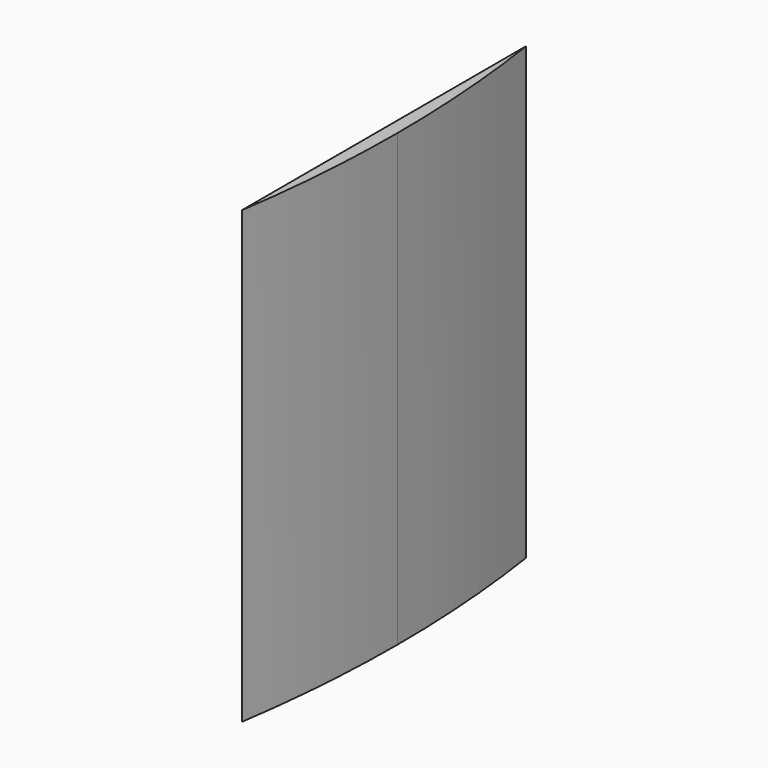
from build123d import *

# Parameters (mm, degrees)
F1_DEPTH = 25


with BuildPart() as f1:
    # F0 (on Top) → F1 (new body)
    with BuildSketch(Plane.XY):
        with BuildLine():
            ThreePointArc((69.0609236135, -14.071139842), (69.6167826315, -9.1510956185), (69.8024168807, -4.2032320052))
            ThreePointArc((69.8024168807, -4.2032320052), (69.6167826315, 0.744631608), (69.0609236135, 5.6646758315))
            Line((69.0609236135, 5.6646758315), (69.0609236135, -14.071139842))
        make_face()
    extrude(amount=F1_DEPTH)


solid = f1.part
